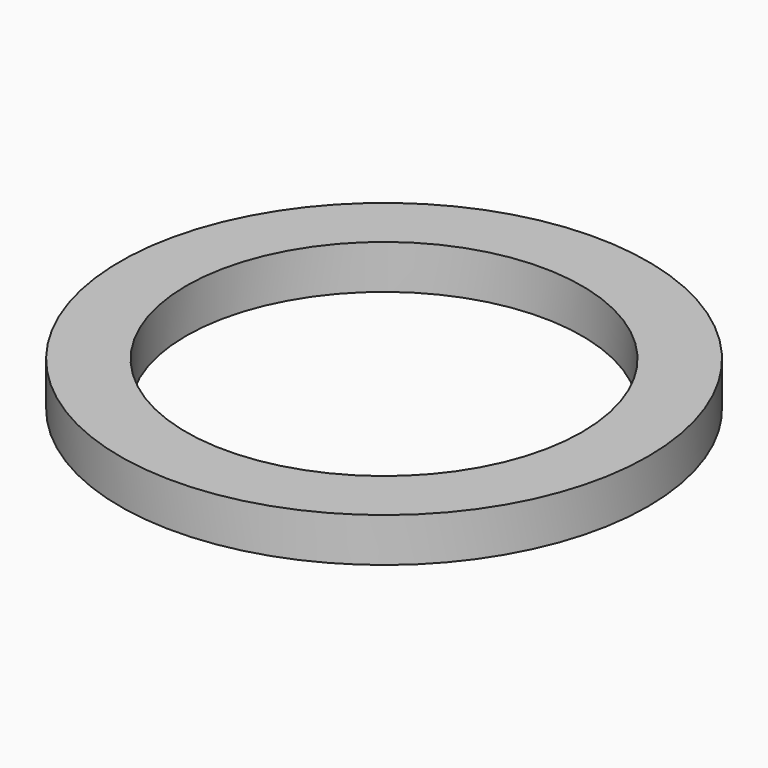
from build123d import *

# Parameters (mm, degrees)
F0_R     = 120
F0_R_2   = 90
F1_DEPTH = 20


# Not quite as in the source:
# - a feature of the source that left no trace in its solid (it failed there, or was rolled back) is left out


with BuildPart() as f1:
    # F0 (on Top) → F1 (new body)
    with BuildSketch(Plane.XY):
        Circle(F0_R)
        Circle(F0_R_2, mode=Mode.SUBTRACT)
    extrude(amount=F1_DEPTH)


solid = f1.part
